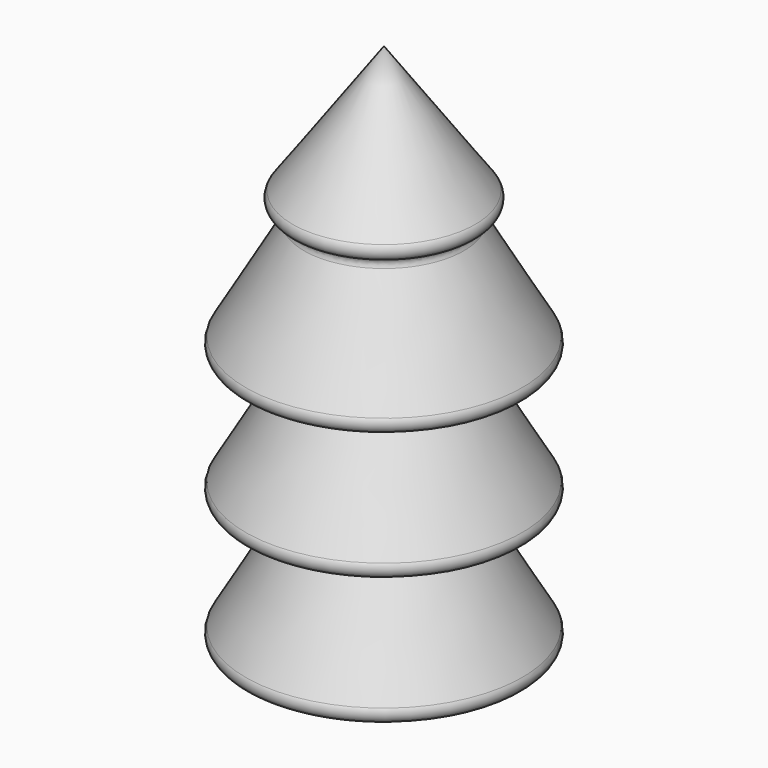
from build123d import *

# Parameters (mm, degrees)
F2_R = 1.778
F3_R = 1.27


# Not quite as in the source:
# - a feature names something its author has since deleted; it is built from what else it names


with BuildPart() as f1:
    # F0 (on Front) → F1 (revolve)
    with BuildSketch(Plane.XZ):
        Polygon((-25.4, -34.3397652524), (0, -34.3397652524), (0, 56.4082281518), (-17.78, 31.651370516), (-12.7, 31.651370516), (-25.4, 9.6543252599), (-12.7, 9.6543252599), (-25.4, -12.3427199963), (-12.7, -12.3427199963), align=None)
    revolve(axis=Axis((0, 0, 11.0342314497), (0, 0, -1)))

    # F2
    f2_edges = [f1.edges().sort_by_distance(p)[0] for p in [
        (17.78, 0, 31.651371),
        (25.4, 0, 9.654325),
        (25.4, 0, -12.34272),
        (25.4, 0, -34.339765),
    ]]
    fillet(f2_edges, radius=F2_R)

    # F3
    f3_edges = [f1.edges().sort_by_distance(p)[0] for p in [
        (12.7, 0, 31.651371),
        (12.7, 0, -12.34272),
        (12.7, 0, 9.654325),
    ]]
    fillet(f3_edges, radius=F3_R)


solid = f1.part
